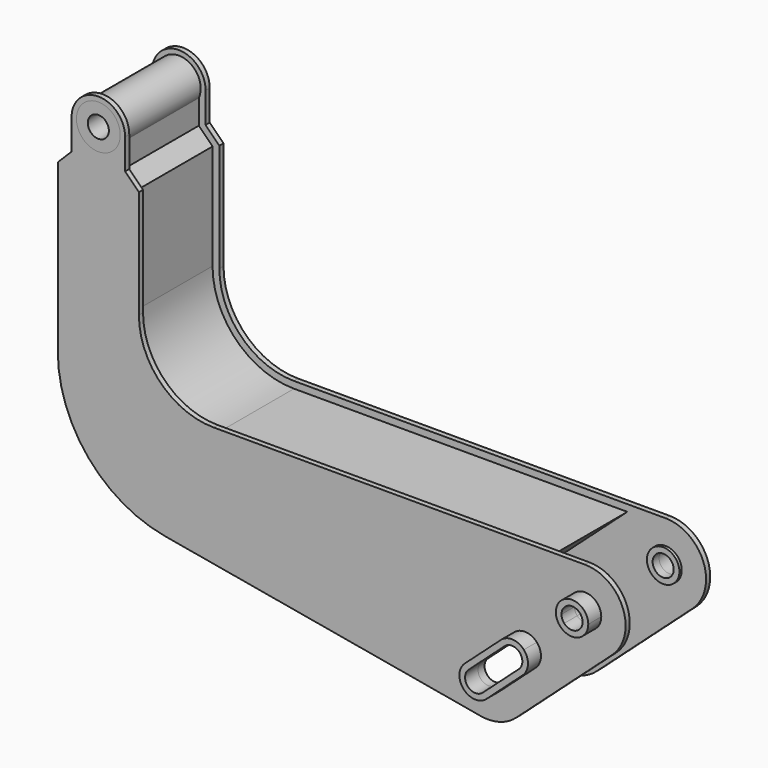
from build123d import *

# Parameters (mm, degrees)
F0_R          = 67.5
F0_R_2        = 100
F0_R_3        = 50
F1_DEPTH      = 16
F3_R          = 67.5
F4_DEPTH      = 16
F0_R_4        = 32.5
F6_DEPTH      = 25
F6_DEPTH_BACK = 50
F3_R_2        = 50
F3_R_3        = 32.5
F7_DEPTH      = 326
F8_DEPTH      = 294
F9_DEPTH      = 50
F9_DEPTH_BACK = 25


# Not quite as in the source:
# - a feature names something its author has since deleted; it is built from what else it names


with BuildPart() as f1:
    # F0 (on Front) → F1 (new body)
    with BuildSketch(Plane.XZ):
        with BuildLine():
            ThreePointArc((-82.5, 0), (0, -82.5), (82.5, 0))
            ThreePointArc((82.5, 0), (0, 82.5), (-82.5, 0))
        make_face()
        Circle(F0_R, mode=Mode.SUBTRACT)
        with BuildLine():
            Line((82.5, -94.1278237248), (82.5, 0))
            ThreePointArc((82.5, 0), (0, -82.5), (-82.5, 0))
            Line((-82.5, 0), (-82.5, -94.1278237248))
            Line((-82.5, -94.1278237248), (-125, -136.6278237248))
            Line((-125, -136.6278237248), (-125, -649.8239662293))
            ThreePointArc((-125, -649.8239662293), (-31.4177772476, -906.9390101039), (205.5407289332, -1043.7470674342))
            Line((205.5407289332, -1043.7470674342), (1178.6344334276, -1215.3297422941))
            ThreePointArc((1178.6344334276, -1215.3297422941), (1237.0415527805, -1212.2687548745), (1288.1956753509, -1183.9135617146))
            Line((1288.1956753509, -1183.9135617146), (1583.6413257949, -917.8931031847))
            ThreePointArc((1583.6413257949, -917.8931031847), (1616.6975533122, -780.2040063068), (1500, -700))
            Line((1500, -700), (355, -700))
            ThreePointArc((355, -700), (192.3654403271, -632.6345596729), (125, -470))
            Line((125, -470), (125, -136.6278237248))
            Line((125, -136.6278237248), (82.5, -94.1278237248))
        make_face()
        with BuildLine():
            Line((1135.8290091732, -1018.3377599958), (1247.3007329948, -917.968169042))
            ThreePointArc((1247.3007329948, -917.968169042), (1388.5282761784, -925.3695909538), (1381.1268542665, -1066.5971341375))
            Line((1381.1268542665, -1066.5971341375), (1269.6551304449, -1166.9667250913))
            ThreePointArc((1269.6551304449, -1166.9667250913), (1128.4275872613, -1159.5653031794), (1135.8290091732, -1018.3377599958))
        make_face(mode=Mode.SUBTRACT)
        with Locations((1500, -825)):
            Circle(F0_R_2, mode=Mode.SUBTRACT)
        with Locations((1500, -825)):
            Circle(F0_R_2)
        with Locations((1500, -825)):
            Circle(F0_R_3, mode=Mode.SUBTRACT)
        with BuildLine():
            ThreePointArc((1381.1268542665, -1066.5971341375), (1388.5282761784, -925.3695909538), (1247.3007329948, -917.968169042))
            Line((1247.3007329948, -917.968169042), (1135.8290091732, -1018.3377599958))
            ThreePointArc((1135.8290091732, -1018.3377599958), (1128.4275872613, -1159.5653031794), (1269.6551304449, -1166.9667250913))
            Line((1269.6551304449, -1166.9667250913), (1381.1268542665, -1066.5971341375))
        make_face()
        with BuildLine():
            Line((1169.2855394911, -1055.4950012697), (1280.7572633127, -955.1254103158))
            ThreePointArc((1280.7572633127, -955.1254103158), (1351.3710349045, -958.8261212718), (1347.6703239486, -1029.4398928636))
            Line((1347.6703239486, -1029.4398928636), (1236.198600127, -1129.8094838174))
            ThreePointArc((1236.198600127, -1129.8094838174), (1165.5848285352, -1126.1087728615), (1169.2855394911, -1055.4950012697))
        make_face(mode=Mode.SUBTRACT)
    extrude(amount=F1_DEPTH)

    # F0 (on Front) → F6 (join, two sides)
    with BuildSketch(Plane.XZ) as f6_sk:
        with Locations((1500, -825)):
            Circle(F0_R_3)
        with Locations((1500, -825)):
            Circle(F0_R_4, mode=Mode.SUBTRACT)
        with BuildLine():
            ThreePointArc((1347.6703239486, -1029.4398928636), (1351.3710349045, -958.8261212718), (1280.7572633127, -955.1254103158))
            Line((1280.7572633127, -955.1254103158), (1169.2855394911, -1055.4950012697))
            ThreePointArc((1169.2855394911, -1055.4950012697), (1165.5848285352, -1126.1087728615), (1236.198600127, -1129.8094838174))
            Line((1236.198600127, -1129.8094838174), (1347.6703239486, -1029.4398928636))
        make_face()
        with BuildLine():
            ThreePointArc((1292.467048924, -968.1304447617), (1338.3660004587, -970.5359068831), (1335.9605383373, -1016.4348584177))
            Line((1335.9605383373, -1016.4348584177), (1224.4888145157, -1116.8044493716))
            ThreePointArc((1224.4888145157, -1116.8044493716), (1178.589862981, -1114.3989872502), (1180.9953251024, -1068.5000357155))
            Line((1180.9953251024, -1068.5000357155), (1292.467048924, -968.1304447617))
        make_face(mode=Mode.SUBTRACT)
    extrude(amount=F6_DEPTH)
    extrude(f6_sk.sketch, amount=-F6_DEPTH_BACK)


with BuildPart() as f4:
    # F3 (on offset) → F4 (new body)
    with BuildSketch(Plane.XZ.offset(326)):
        with BuildLine():
            Line((82.5, -94.1278237248), (82.5, 0))
            ThreePointArc((82.5, 0), (0, -82.5), (-82.5, 0))
            Line((-82.5, 0), (-82.5, -94.1278237248))
            Line((-82.5, -94.1278237248), (-125, -136.6278237248))
            Line((-125, -136.6278237248), (-125, -649.8239662293))
            ThreePointArc((-125, -649.8239662293), (-31.4177772476, -906.9390101039), (205.5407289332, -1043.7470674342))
            Line((205.5407289332, -1043.7470674342), (1178.6344334276, -1215.3297422941))
            ThreePointArc((1178.6344334276, -1215.3297422941), (1237.0415527805, -1212.2687548745), (1288.1956753509, -1183.9135617146))
            Line((1288.1956753509, -1183.9135617146), (1583.6413257949, -917.8931031847))
            ThreePointArc((1583.6413257949, -917.8931031847), (1616.6975533122, -780.2040063068), (1500, -700))
            Line((1500, -700), (355, -700))
            ThreePointArc((355, -700), (192.3654403271, -632.6345596729), (125, -470))
            Line((125, -470), (125, -136.6278237248))
            Line((125, -136.6278237248), (82.5, -94.1278237248))
        make_face()
        with BuildLine():
            ThreePointArc((1247.3007329948, -917.968169042), (1319.4473892549, -892.4196981143), (1388.5282761784, -925.3695909538))
            ThreePointArc((1388.5282761784, -925.3695909538), (1414.0767471061, -997.516247214), (1381.1268542665, -1066.5971341375))
            Line((1381.1268542665, -1066.5971341375), (1269.6551304449, -1166.9667250913))
            ThreePointArc((1269.6551304449, -1166.9667250913), (1128.4275872613, -1159.5653031794), (1135.8290091732, -1018.3377599958))
            Line((1135.8290091732, -1018.3377599958), (1247.3007329948, -917.968169042))
        make_face(mode=Mode.SUBTRACT)
        with BuildLine():
            ThreePointArc((1425.6855174523, -891.9130606359), (1406.6419573503, -860.8367949545), (1400, -825))
            ThreePointArc((1400, -825), (1500, -725), (1600, -825))
            ThreePointArc((1600, -825), (1535.8367949545, -918.3580426497), (1425.6855174523, -891.9130606359))
        make_face(mode=Mode.SUBTRACT)
        with BuildLine():
            ThreePointArc((1381.1268542665, -1066.5971341375), (1414.0767471061, -997.516247214), (1388.5282761784, -925.3695909538))
            ThreePointArc((1388.5282761784, -925.3695909538), (1319.4473892549, -892.4196981143), (1247.3007329948, -917.968169042))
            Line((1247.3007329948, -917.968169042), (1135.8290091732, -1018.3377599958))
            ThreePointArc((1135.8290091732, -1018.3377599958), (1128.4275872613, -1159.5653031794), (1269.6551304449, -1166.9667250913))
            Line((1269.6551304449, -1166.9667250913), (1381.1268542665, -1066.5971341375))
        make_face()
        with BuildLine():
            ThreePointArc((1280.7572633127, -955.1254103158), (1316.8305914428, -942.351174852), (1351.3710349045, -958.8261212718))
            ThreePointArc((1351.3710349045, -958.8261212718), (1364.1452703684, -994.8994494019), (1347.6703239486, -1029.4398928636))
            Line((1347.6703239486, -1029.4398928636), (1236.198600127, -1129.8094838174))
            ThreePointArc((1236.198600127, -1129.8094838174), (1165.5848285352, -1126.1087728615), (1169.2855394911, -1055.4950012697))
            Line((1169.2855394911, -1055.4950012697), (1280.7572633127, -955.1254103158))
        make_face(mode=Mode.SUBTRACT)
        with BuildLine():
            ThreePointArc((-82.5, 0), (0, -82.5), (82.5, 0))
            ThreePointArc((82.5, 0), (0, 82.5), (-82.5, 0))
        make_face()
        Circle(F3_R, mode=Mode.SUBTRACT)
        with BuildLine():
            Line((1400, -825), (1450, -825))
            ThreePointArc((1450, -825), (1500, -775), (1550, -825))
            ThreePointArc((1550, -825), (1517.9183974773, -871.6790213249), (1462.8427587261, -858.4565303179))
            Line((1462.8427587261, -858.4565303179), (1425.6855174523, -891.9130606359))
            ThreePointArc((1425.6855174523, -891.9130606359), (1535.8367949545, -918.3580426497), (1600, -825))
            ThreePointArc((1600, -825), (1500, -725), (1400, -825))
        make_face()
        with BuildLine():
            ThreePointArc((1462.8427587261, -858.4565303179), (1453.3209786751, -842.9183974773), (1450, -825))
            Line((1450, -825), (1400, -825))
            ThreePointArc((1400, -825), (1406.6419573503, -860.8367949545), (1425.6855174523, -891.9130606359))
            Line((1425.6855174523, -891.9130606359), (1462.8427587261, -858.4565303179))
        make_face()
    extrude(amount=-F4_DEPTH)

    # F3 (on offset) → F9 (join, two sides)
    with BuildSketch(Plane.XZ.offset(326)) as f9_sk:
        with BuildLine():
            ThreePointArc((1467.5, -825), (1500, -792.5), (1532.5, -825))
            ThreePointArc((1532.5, -825), (1511.6469583602, -855.3413638612), (1475.847793172, -846.7467447067))
            Line((1475.847793172, -846.7467447067), (1462.8427587261, -858.4565303179))
            ThreePointArc((1462.8427587261, -858.4565303179), (1517.9183974773, -871.6790213249), (1550, -825))
            ThreePointArc((1550, -825), (1500, -775), (1450, -825))
            Line((1450, -825), (1467.5, -825))
        make_face()
        with BuildLine():
            ThreePointArc((1475.847793172, -846.7467447067), (1469.6586361388, -836.6469583602), (1467.5, -825))
            Line((1467.5, -825), (1450, -825))
            ThreePointArc((1450, -825), (1453.3209786751, -842.9183974773), (1462.8427587261, -858.4565303179))
            Line((1462.8427587261, -858.4565303179), (1475.847793172, -846.7467447067))
        make_face()
        with BuildLine():
            ThreePointArc((1347.6703239486, -1029.4398928636), (1364.1452703684, -994.8994494019), (1351.3710349045, -958.8261212718))
            ThreePointArc((1351.3710349045, -958.8261212718), (1316.8305914428, -942.351174852), (1280.7572633127, -955.1254103158))
            Line((1280.7572633127, -955.1254103158), (1169.2855394911, -1055.4950012697))
            ThreePointArc((1169.2855394911, -1055.4950012697), (1165.5848285352, -1126.1087728615), (1236.198600127, -1129.8094838174))
            Line((1236.198600127, -1129.8094838174), (1347.6703239486, -1029.4398928636))
        make_face()
        with BuildLine():
            ThreePointArc((1292.467048924, -968.1304447617), (1315.9147122085, -959.8271917102), (1338.3660004587, -970.5359068831))
            ThreePointArc((1338.3660004587, -970.5359068831), (1346.6692535102, -993.9835701676), (1335.9605383373, -1016.4348584177))
            Line((1335.9605383373, -1016.4348584177), (1224.4888145157, -1116.8044493716))
            ThreePointArc((1224.4888145157, -1116.8044493716), (1178.589862981, -1114.3989872502), (1180.9953251024, -1068.5000357155))
            Line((1180.9953251024, -1068.5000357155), (1292.467048924, -968.1304447617))
        make_face(mode=Mode.SUBTRACT)
    extrude(amount=F9_DEPTH)
    extrude(f9_sk.sketch, amount=-F9_DEPTH_BACK)


with BuildPart() as f7:
    # F3 (on offset) → F7 (new body, through all)
    with BuildSketch(Plane.XZ.offset(326)):
        Circle(F3_R)
        Circle(F3_R_2, mode=Mode.SUBTRACT)
        Circle(F3_R_2)
        Circle(F3_R_3, mode=Mode.SUBTRACT)
    extrude(amount=-F7_DEPTH)


with BuildPart() as f8:
    # F5 (on face) → F8 (new body, through all)
    with BuildSketch(Plane.XZ.offset(16)):
        with BuildLine():
            Line((61.5, -102.8263085346), (61.5, -27.8208554865))
            ThreePointArc((61.5, -27.8208554865), (0, -67.5), (-61.5, -27.8208554865))
            Line((-61.5, -27.8208554865), (-61.5, -102.8263085346))
            Line((-61.5, -102.8263085346), (-104, -145.3263085346))
            Line((-104, -145.3263085346), (-104, -649.8239662293))
            ThreePointArc((-104, -649.8239662293), (-15.3308439421, -893.4404703005), (209.1873406642, -1023.0661046209))
            Line((209.1873406642, -1023.0661046209), (909.7041001333, -1146.5861097538))
            Line((909.7041001333, -1146.5861097538), (1382.3653597634, -721))
            Line((1382.3653597634, -721), (355, -721))
            ThreePointArc((355, -721), (177.5161979222, -647.4838020778), (104, -470))
            Line((104, -470), (104, -145.3263085346))
            Line((104, -145.3263085346), (61.5, -102.8263085346))
        make_face()
    extrude(amount=F8_DEPTH)


solid = Compound([f1.part, f4.part, f7.part, f8.part])
